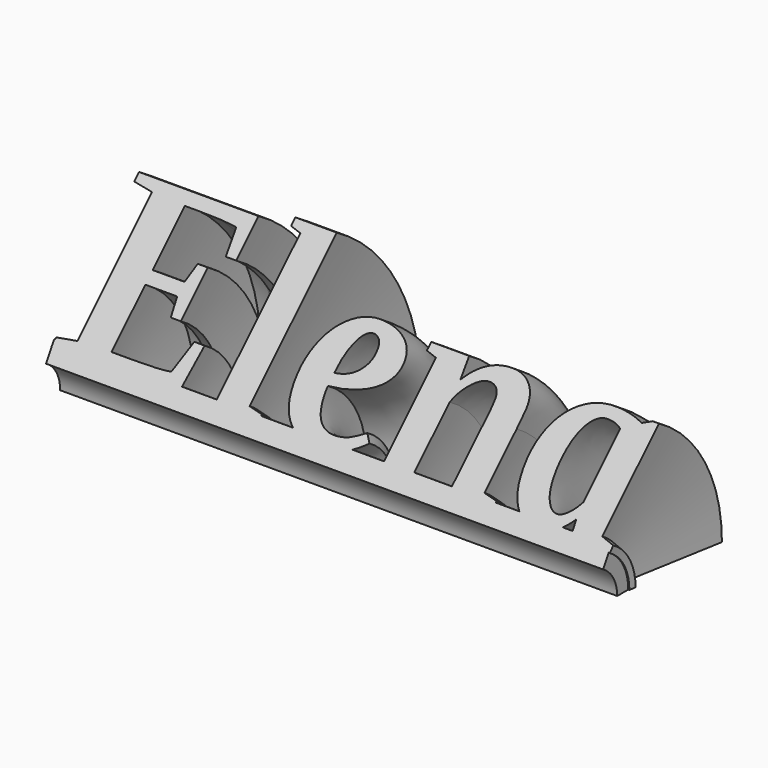
from build123d import *

# Parameters (mm, degrees)
F0_TEXT_SIZE = 40.9210307731
F1_W         = 98.1203764677
F1_H         = 3.5139527172
F3_ANGLE     = 60


# Not quite as in the source:
# - Text() gives the source's letters only with a copy of the font that has no kerning and outlines rounded to 1/6400 em; it was checked with that copy


with BuildPart() as f3:
    # F0 (on Top) + F1 (on Top) → F3 (revolve)
    with BuildSketch(Plane.XY):
        with Locations((-76.4284729958, -12.907018885)):
            Text('Elena', F0_TEXT_SIZE, font='Tinos', font_style=FontStyle.BOLDITALIC, text_align=(TextAlign.LEFT, TextAlign.BOTTOM))
    with BuildSketch(Plane.XY):
        with Locations((-27.638591826, -13.5827790946)):
            Rectangle(F1_W, F1_H)
    revolve(axis=Axis((-26.827679947, -21.5567499399, 0), (1, 0, 0)), revolution_arc=F3_ANGLE)


solid = f3.part
